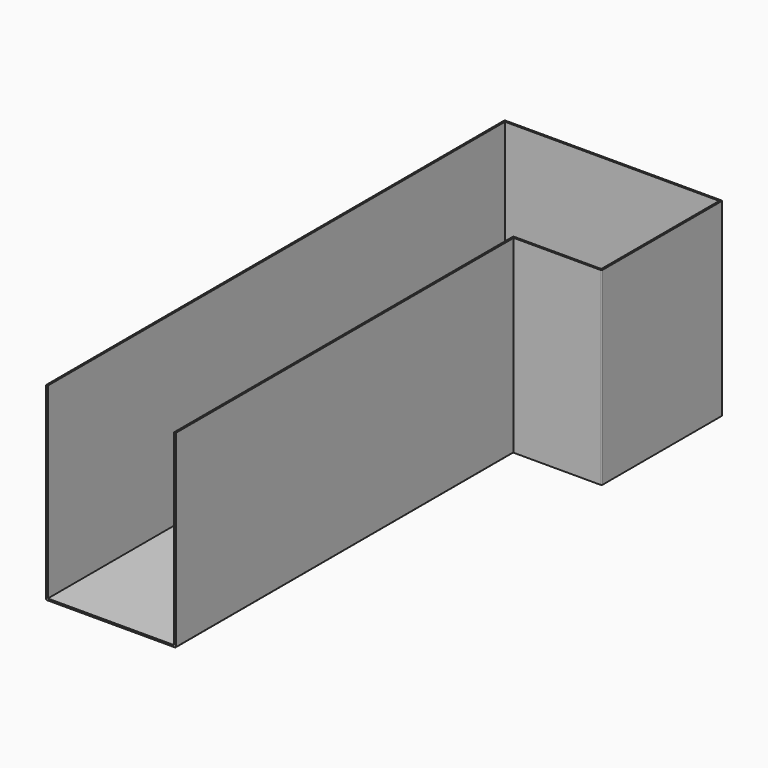
from build123d import *

# Parameters (mm, degrees)
F1_DEPTH = 426
F3_DEPTH = 4
F4_R     = 2


# Not quite as in the source:
# - a feature names something its author has since deleted; it is built from what else it names


with BuildPart() as f1:
    # F0 (on Top) → F1 (new body)
    with BuildSketch(Plane.XY):
        Polygon((-200, -343), (0, -343), (0, 0), (-495, 0), (-495, -1303), (-491, -1303), (-491, -4), (-4, -4), (-4, -339), (-204, -339), (-204, -1303), (-200, -1303), align=None)
    extrude(amount=F1_DEPTH)

    # F2 (on Top) → F3 (join)
    with BuildSketch(Plane.XY):
        Polygon((0, 0), (-495, 0), (-495, -1303), (-200, -1303), (-200, -343), (0, -343), align=None)
    extrude(amount=-F3_DEPTH)

    # F4
    f4_edges = [f1.edges().sort_by_distance(p)[0] for p in [
        (-200, -823, -4),
        (-495, -651.5, -4),
        (-247.5, 0, -4),
        (-495, 0, 211),
        (0, -343, 211),
        (0, 0, 211),
    ]]
    fillet(f4_edges, radius=F4_R)


solid = f1.part
